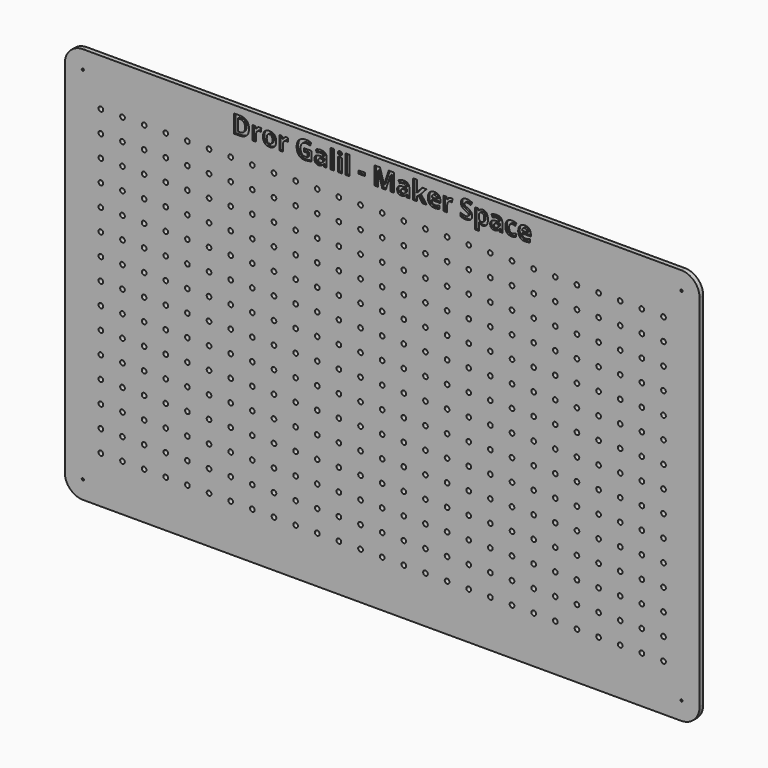
from build123d import *

# Parameters (mm, degrees)
F0_W         = 880
F0_H         = 550
F0_R         = 3.25
F1_DEPTH     = 6.35
F2_R         = 1.5
F3_DEPTH     = 25
F4_R         = 25.4
F5_TEXT_SIZE = 34.7222222222
F6_DEPTH     = 2.54


# Not quite as in the source:
# - Text() gives the source's letters only with a copy of the font that has no kerning and outlines rounded to 1/6400 em; it was checked with that copy


with BuildPart() as f1:
    # F0 (on Front) → F1 (new body)
    with BuildSketch(Plane.XZ):
        Rectangle(F0_W, F0_H)
        with Locations((-390, -210)):
            Circle(F0_R, mode=Mode.SUBTRACT)
        with Locations((-360, -210)):
            Circle(F0_R, mode=Mode.SUBTRACT)
        with Locations((-330, -210)):
            Circle(F0_R, mode=Mode.SUBTRACT)
        with Locations((-300, -210)):
            Circle(F0_R, mode=Mode.SUBTRACT)
        with Locations((-270, -210)):
            Circle(F0_R, mode=Mode.SUBTRACT)
        with Locations((-240, -210)):
            Circle(F0_R, mode=Mode.SUBTRACT)
        with Locations((-390, -180)):
            Circle(F0_R, mode=Mode.SUBTRACT)
        with Locations((-360, -180)):
            Circle(F0_R, mode=Mode.SUBTRACT)
        with Locations((-390, -150)):
            Circle(F0_R, mode=Mode.SUBTRACT)
        with Locations((-360, -150)):
            Circle(F0_R, mode=Mode.SUBTRACT)
        with Locations((-330, -180)):
            Circle(F0_R, mode=Mode.SUBTRACT)
        with Locations((-300, -180)):
            Circle(F0_R, mode=Mode.SUBTRACT)
        with Locations((-270, -180)):
            Circle(F0_R, mode=Mode.SUBTRACT)
        with Locations((-240, -180)):
            Circle(F0_R, mode=Mode.SUBTRACT)
        with Locations((-330, -150)):
            Circle(F0_R, mode=Mode.SUBTRACT)
        with Locations((-300, -150)):
            Circle(F0_R, mode=Mode.SUBTRACT)
        with Locations((-270, -150)):
            Circle(F0_R, mode=Mode.SUBTRACT)
        with Locations((-240, -150)):
            Circle(F0_R, mode=Mode.SUBTRACT)
        with Locations((-210, -210)):
            Circle(F0_R, mode=Mode.SUBTRACT)
        with Locations((-180, -210)):
            Circle(F0_R, mode=Mode.SUBTRACT)
        with Locations((-150, -210)):
            Circle(F0_R, mode=Mode.SUBTRACT)
        with Locations((-120, -210)):
            Circle(F0_R, mode=Mode.SUBTRACT)
        with Locations((-90, -210)):
            Circle(F0_R, mode=Mode.SUBTRACT)
        with Locations((-60, -210)):
            Circle(F0_R, mode=Mode.SUBTRACT)
        with Locations((-30, -210)):
            Circle(F0_R, mode=Mode.SUBTRACT)
        with Locations((-210, -180)):
            Circle(F0_R, mode=Mode.SUBTRACT)
        with Locations((-180, -180)):
            Circle(F0_R, mode=Mode.SUBTRACT)
        with Locations((-150, -180)):
            Circle(F0_R, mode=Mode.SUBTRACT)
        with Locations((-120, -180)):
            Circle(F0_R, mode=Mode.SUBTRACT)
        with Locations((-210, -150)):
            Circle(F0_R, mode=Mode.SUBTRACT)
        with Locations((-180, -150)):
            Circle(F0_R, mode=Mode.SUBTRACT)
        with Locations((-150, -150)):
            Circle(F0_R, mode=Mode.SUBTRACT)
        with Locations((-120, -150)):
            Circle(F0_R, mode=Mode.SUBTRACT)
        with Locations((-90, -180)):
            Circle(F0_R, mode=Mode.SUBTRACT)
        with Locations((-60, -180)):
            Circle(F0_R, mode=Mode.SUBTRACT)
        with Locations((-30, -180)):
            Circle(F0_R, mode=Mode.SUBTRACT)
        with Locations((-90, -150)):
            Circle(F0_R, mode=Mode.SUBTRACT)
        with Locations((-60, -150)):
            Circle(F0_R, mode=Mode.SUBTRACT)
        with Locations((-30, -150)):
            Circle(F0_R, mode=Mode.SUBTRACT)
        with Locations((-390, -120)):
            Circle(F0_R, mode=Mode.SUBTRACT)
        with Locations((-360, -120)):
            Circle(F0_R, mode=Mode.SUBTRACT)
        with Locations((-390, -90)):
            Circle(F0_R, mode=Mode.SUBTRACT)
        with Locations((-360, -90)):
            Circle(F0_R, mode=Mode.SUBTRACT)
        with Locations((-330, -120)):
            Circle(F0_R, mode=Mode.SUBTRACT)
        with Locations((-300, -120)):
            Circle(F0_R, mode=Mode.SUBTRACT)
        with Locations((-270, -120)):
            Circle(F0_R, mode=Mode.SUBTRACT)
        with Locations((-240, -120)):
            Circle(F0_R, mode=Mode.SUBTRACT)
        with Locations((-330, -90)):
            Circle(F0_R, mode=Mode.SUBTRACT)
        with Locations((-300, -90)):
            Circle(F0_R, mode=Mode.SUBTRACT)
        with Locations((-270, -90)):
            Circle(F0_R, mode=Mode.SUBTRACT)
        with Locations((-240, -90)):
            Circle(F0_R, mode=Mode.SUBTRACT)
        with Locations((-390, -60)):
            Circle(F0_R, mode=Mode.SUBTRACT)
        with Locations((-360, -60)):
            Circle(F0_R, mode=Mode.SUBTRACT)
        with Locations((-390, -30)):
            Circle(F0_R, mode=Mode.SUBTRACT)
        with Locations((-360, -30)):
            Circle(F0_R, mode=Mode.SUBTRACT)
        with Locations((-330, -60)):
            Circle(F0_R, mode=Mode.SUBTRACT)
        with Locations((-300, -60)):
            Circle(F0_R, mode=Mode.SUBTRACT)
        with Locations((-270, -60)):
            Circle(F0_R, mode=Mode.SUBTRACT)
        with Locations((-240, -60)):
            Circle(F0_R, mode=Mode.SUBTRACT)
        with Locations((-330, -30)):
            Circle(F0_R, mode=Mode.SUBTRACT)
        with Locations((-300, -30)):
            Circle(F0_R, mode=Mode.SUBTRACT)
        with Locations((-270, -30)):
            Circle(F0_R, mode=Mode.SUBTRACT)
        with Locations((-240, -30)):
            Circle(F0_R, mode=Mode.SUBTRACT)
        with Locations((-210, -120)):
            Circle(F0_R, mode=Mode.SUBTRACT)
        with Locations((-180, -120)):
            Circle(F0_R, mode=Mode.SUBTRACT)
        with Locations((-150, -120)):
            Circle(F0_R, mode=Mode.SUBTRACT)
        with Locations((-120, -120)):
            Circle(F0_R, mode=Mode.SUBTRACT)
        with Locations((-210, -90)):
            Circle(F0_R, mode=Mode.SUBTRACT)
        with Locations((-180, -90)):
            Circle(F0_R, mode=Mode.SUBTRACT)
        with Locations((-150, -90)):
            Circle(F0_R, mode=Mode.SUBTRACT)
        with Locations((-120, -90)):
            Circle(F0_R, mode=Mode.SUBTRACT)
        with Locations((-90, -120)):
            Circle(F0_R, mode=Mode.SUBTRACT)
        with Locations((-60, -120)):
            Circle(F0_R, mode=Mode.SUBTRACT)
        with Locations((-30, -120)):
            Circle(F0_R, mode=Mode.SUBTRACT)
        with Locations((-90, -90)):
            Circle(F0_R, mode=Mode.SUBTRACT)
        with Locations((-60, -90)):
            Circle(F0_R, mode=Mode.SUBTRACT)
        with Locations((-30, -90)):
            Circle(F0_R, mode=Mode.SUBTRACT)
        with Locations((-210, -60)):
            Circle(F0_R, mode=Mode.SUBTRACT)
        with Locations((-180, -60)):
            Circle(F0_R, mode=Mode.SUBTRACT)
        with Locations((-150, -60)):
            Circle(F0_R, mode=Mode.SUBTRACT)
        with Locations((-120, -60)):
            Circle(F0_R, mode=Mode.SUBTRACT)
        with Locations((-210, -30)):
            Circle(F0_R, mode=Mode.SUBTRACT)
        with Locations((-180, -30)):
            Circle(F0_R, mode=Mode.SUBTRACT)
        with Locations((-150, -30)):
            Circle(F0_R, mode=Mode.SUBTRACT)
        with Locations((-120, -30)):
            Circle(F0_R, mode=Mode.SUBTRACT)
        with Locations((-90, -60)):
            Circle(F0_R, mode=Mode.SUBTRACT)
        with Locations((-60, -60)):
            Circle(F0_R, mode=Mode.SUBTRACT)
        with Locations((-30, -60)):
            Circle(F0_R, mode=Mode.SUBTRACT)
        with Locations((-90, -30)):
            Circle(F0_R, mode=Mode.SUBTRACT)
        with Locations((-60, -30)):
            Circle(F0_R, mode=Mode.SUBTRACT)
        with Locations((-30, -30)):
            Circle(F0_R, mode=Mode.SUBTRACT)
        with Locations((0, -210)):
            Circle(F0_R, mode=Mode.SUBTRACT)
        with Locations((30, -210)):
            Circle(F0_R, mode=Mode.SUBTRACT)
        with Locations((60, -210)):
            Circle(F0_R, mode=Mode.SUBTRACT)
        with Locations((90, -210)):
            Circle(F0_R, mode=Mode.SUBTRACT)
        with Locations((120, -210)):
            Circle(F0_R, mode=Mode.SUBTRACT)
        with Locations((150, -210)):
            Circle(F0_R, mode=Mode.SUBTRACT)
        with Locations((180, -210)):
            Circle(F0_R, mode=Mode.SUBTRACT)
        with Locations((210, -210)):
            Circle(F0_R, mode=Mode.SUBTRACT)
        with Locations((0, -180)):
            Circle(F0_R, mode=Mode.SUBTRACT)
        with Locations((30, -180)):
            Circle(F0_R, mode=Mode.SUBTRACT)
        with Locations((60, -180)):
            Circle(F0_R, mode=Mode.SUBTRACT)
        with Locations((90, -180)):
            Circle(F0_R, mode=Mode.SUBTRACT)
        with Locations((0, -150)):
            Circle(F0_R, mode=Mode.SUBTRACT)
        with Locations((30, -150)):
            Circle(F0_R, mode=Mode.SUBTRACT)
        with Locations((60, -150)):
            Circle(F0_R, mode=Mode.SUBTRACT)
        with Locations((90, -150)):
            Circle(F0_R, mode=Mode.SUBTRACT)
        with Locations((120, -180)):
            Circle(F0_R, mode=Mode.SUBTRACT)
        with Locations((150, -180)):
            Circle(F0_R, mode=Mode.SUBTRACT)
        with Locations((180, -180)):
            Circle(F0_R, mode=Mode.SUBTRACT)
        with Locations((210, -180)):
            Circle(F0_R, mode=Mode.SUBTRACT)
        with Locations((120, -150)):
            Circle(F0_R, mode=Mode.SUBTRACT)
        with Locations((150, -150)):
            Circle(F0_R, mode=Mode.SUBTRACT)
        with Locations((180, -150)):
            Circle(F0_R, mode=Mode.SUBTRACT)
        with Locations((210, -150)):
            Circle(F0_R, mode=Mode.SUBTRACT)
        with Locations((240, -210)):
            Circle(F0_R, mode=Mode.SUBTRACT)
        with Locations((270, -210)):
            Circle(F0_R, mode=Mode.SUBTRACT)
        with Locations((300, -210)):
            Circle(F0_R, mode=Mode.SUBTRACT)
        with Locations((330, -210)):
            Circle(F0_R, mode=Mode.SUBTRACT)
        with Locations((360, -210)):
            Circle(F0_R, mode=Mode.SUBTRACT)
        with Locations((390, -210)):
            Circle(F0_R, mode=Mode.SUBTRACT)
        with Locations((240, -180)):
            Circle(F0_R, mode=Mode.SUBTRACT)
        with Locations((270, -180)):
            Circle(F0_R, mode=Mode.SUBTRACT)
        with Locations((300, -180)):
            Circle(F0_R, mode=Mode.SUBTRACT)
        with Locations((240, -150)):
            Circle(F0_R, mode=Mode.SUBTRACT)
        with Locations((270, -150)):
            Circle(F0_R, mode=Mode.SUBTRACT)
        with Locations((300, -150)):
            Circle(F0_R, mode=Mode.SUBTRACT)
        with Locations((330, -180)):
            Circle(F0_R, mode=Mode.SUBTRACT)
        with Locations((360, -180)):
            Circle(F0_R, mode=Mode.SUBTRACT)
        with Locations((390, -180)):
            Circle(F0_R, mode=Mode.SUBTRACT)
        with Locations((330, -150)):
            Circle(F0_R, mode=Mode.SUBTRACT)
        with Locations((360, -150)):
            Circle(F0_R, mode=Mode.SUBTRACT)
        with Locations((390, -150)):
            Circle(F0_R, mode=Mode.SUBTRACT)
        with Locations((0, -120)):
            Circle(F0_R, mode=Mode.SUBTRACT)
        with Locations((30, -120)):
            Circle(F0_R, mode=Mode.SUBTRACT)
        with Locations((60, -120)):
            Circle(F0_R, mode=Mode.SUBTRACT)
        with Locations((90, -120)):
            Circle(F0_R, mode=Mode.SUBTRACT)
        with Locations((0, -90)):
            Circle(F0_R, mode=Mode.SUBTRACT)
        with Locations((30, -90)):
            Circle(F0_R, mode=Mode.SUBTRACT)
        with Locations((60, -90)):
            Circle(F0_R, mode=Mode.SUBTRACT)
        with Locations((90, -90)):
            Circle(F0_R, mode=Mode.SUBTRACT)
        with Locations((120, -120)):
            Circle(F0_R, mode=Mode.SUBTRACT)
        with Locations((150, -120)):
            Circle(F0_R, mode=Mode.SUBTRACT)
        with Locations((180, -120)):
            Circle(F0_R, mode=Mode.SUBTRACT)
        with Locations((210, -120)):
            Circle(F0_R, mode=Mode.SUBTRACT)
        with Locations((120, -90)):
            Circle(F0_R, mode=Mode.SUBTRACT)
        with Locations((150, -90)):
            Circle(F0_R, mode=Mode.SUBTRACT)
        with Locations((180, -90)):
            Circle(F0_R, mode=Mode.SUBTRACT)
        with Locations((210, -90)):
            Circle(F0_R, mode=Mode.SUBTRACT)
        with Locations((0, -60)):
            Circle(F0_R, mode=Mode.SUBTRACT)
        with Locations((30, -60)):
            Circle(F0_R, mode=Mode.SUBTRACT)
        with Locations((60, -60)):
            Circle(F0_R, mode=Mode.SUBTRACT)
        with Locations((90, -60)):
            Circle(F0_R, mode=Mode.SUBTRACT)
        with Locations((0, -30)):
            Circle(F0_R, mode=Mode.SUBTRACT)
        with Locations((30, -30)):
            Circle(F0_R, mode=Mode.SUBTRACT)
        with Locations((60, -30)):
            Circle(F0_R, mode=Mode.SUBTRACT)
        with Locations((90, -30)):
            Circle(F0_R, mode=Mode.SUBTRACT)
        with Locations((120, -60)):
            Circle(F0_R, mode=Mode.SUBTRACT)
        with Locations((150, -60)):
            Circle(F0_R, mode=Mode.SUBTRACT)
        with Locations((180, -60)):
            Circle(F0_R, mode=Mode.SUBTRACT)
        with Locations((210, -60)):
            Circle(F0_R, mode=Mode.SUBTRACT)
        with Locations((120, -30)):
            Circle(F0_R, mode=Mode.SUBTRACT)
        with Locations((150, -30)):
            Circle(F0_R, mode=Mode.SUBTRACT)
        with Locations((180, -30)):
            Circle(F0_R, mode=Mode.SUBTRACT)
        with Locations((210, -30)):
            Circle(F0_R, mode=Mode.SUBTRACT)
        with Locations((240, -120)):
            Circle(F0_R, mode=Mode.SUBTRACT)
        with Locations((270, -120)):
            Circle(F0_R, mode=Mode.SUBTRACT)
        with Locations((300, -120)):
            Circle(F0_R, mode=Mode.SUBTRACT)
        with Locations((240, -90)):
            Circle(F0_R, mode=Mode.SUBTRACT)
        with Locations((270, -90)):
            Circle(F0_R, mode=Mode.SUBTRACT)
        with Locations((300, -90)):
            Circle(F0_R, mode=Mode.SUBTRACT)
        with Locations((330, -120)):
            Circle(F0_R, mode=Mode.SUBTRACT)
        with Locations((360, -120)):
            Circle(F0_R, mode=Mode.SUBTRACT)
        with Locations((390, -120)):
            Circle(F0_R, mode=Mode.SUBTRACT)
        with Locations((330, -90)):
            Circle(F0_R, mode=Mode.SUBTRACT)
        with Locations((360, -90)):
            Circle(F0_R, mode=Mode.SUBTRACT)
        with Locations((390, -90)):
            Circle(F0_R, mode=Mode.SUBTRACT)
        with Locations((240, -60)):
            Circle(F0_R, mode=Mode.SUBTRACT)
        with Locations((270, -60)):
            Circle(F0_R, mode=Mode.SUBTRACT)
        with Locations((300, -60)):
            Circle(F0_R, mode=Mode.SUBTRACT)
        with Locations((240, -30)):
            Circle(F0_R, mode=Mode.SUBTRACT)
        with Locations((270, -30)):
            Circle(F0_R, mode=Mode.SUBTRACT)
        with Locations((300, -30)):
            Circle(F0_R, mode=Mode.SUBTRACT)
        with Locations((330, -60)):
            Circle(F0_R, mode=Mode.SUBTRACT)
        with Locations((360, -60)):
            Circle(F0_R, mode=Mode.SUBTRACT)
        with Locations((390, -60)):
            Circle(F0_R, mode=Mode.SUBTRACT)
        with Locations((330, -30)):
            Circle(F0_R, mode=Mode.SUBTRACT)
        with Locations((360, -30)):
            Circle(F0_R, mode=Mode.SUBTRACT)
        with Locations((390, -30)):
            Circle(F0_R, mode=Mode.SUBTRACT)
        with Locations((-390, 0)):
            Circle(F0_R, mode=Mode.SUBTRACT)
        with Locations((-390, 30)):
            Circle(F0_R, mode=Mode.SUBTRACT)
        with Locations((-360, 0)):
            Circle(F0_R, mode=Mode.SUBTRACT)
        with Locations((-360, 30)):
            Circle(F0_R, mode=Mode.SUBTRACT)
        with Locations((-390, 60)):
            Circle(F0_R, mode=Mode.SUBTRACT)
        with Locations((-360, 60)):
            Circle(F0_R, mode=Mode.SUBTRACT)
        with Locations((-330, 0)):
            Circle(F0_R, mode=Mode.SUBTRACT)
        with Locations((-300, 0)):
            Circle(F0_R, mode=Mode.SUBTRACT)
        with Locations((-330, 30)):
            Circle(F0_R, mode=Mode.SUBTRACT)
        with Locations((-300, 30)):
            Circle(F0_R, mode=Mode.SUBTRACT)
        with Locations((-270, 0)):
            Circle(F0_R, mode=Mode.SUBTRACT)
        with Locations((-240, 0)):
            Circle(F0_R, mode=Mode.SUBTRACT)
        with Locations((-270, 30)):
            Circle(F0_R, mode=Mode.SUBTRACT)
        with Locations((-240, 30)):
            Circle(F0_R, mode=Mode.SUBTRACT)
        with Locations((-330, 60)):
            Circle(F0_R, mode=Mode.SUBTRACT)
        with Locations((-300, 60)):
            Circle(F0_R, mode=Mode.SUBTRACT)
        with Locations((-270, 60)):
            Circle(F0_R, mode=Mode.SUBTRACT)
        with Locations((-240, 60)):
            Circle(F0_R, mode=Mode.SUBTRACT)
        with Locations((-390, 90)):
            Circle(F0_R, mode=Mode.SUBTRACT)
        with Locations((-360, 90)):
            Circle(F0_R, mode=Mode.SUBTRACT)
        with Locations((-390, 120)):
            Circle(F0_R, mode=Mode.SUBTRACT)
        with Locations((-360, 120)):
            Circle(F0_R, mode=Mode.SUBTRACT)
        with Locations((-330, 90)):
            Circle(F0_R, mode=Mode.SUBTRACT)
        with Locations((-300, 90)):
            Circle(F0_R, mode=Mode.SUBTRACT)
        with Locations((-270, 90)):
            Circle(F0_R, mode=Mode.SUBTRACT)
        with Locations((-240, 90)):
            Circle(F0_R, mode=Mode.SUBTRACT)
        with Locations((-330, 120)):
            Circle(F0_R, mode=Mode.SUBTRACT)
        with Locations((-300, 120)):
            Circle(F0_R, mode=Mode.SUBTRACT)
        with Locations((-270, 120)):
            Circle(F0_R, mode=Mode.SUBTRACT)
        with Locations((-240, 120)):
            Circle(F0_R, mode=Mode.SUBTRACT)
        with Locations((-210, 0)):
            Circle(F0_R, mode=Mode.SUBTRACT)
        with Locations((-180, 0)):
            Circle(F0_R, mode=Mode.SUBTRACT)
        with Locations((-210, 30)):
            Circle(F0_R, mode=Mode.SUBTRACT)
        with Locations((-180, 30)):
            Circle(F0_R, mode=Mode.SUBTRACT)
        with Locations((-150, 0)):
            Circle(F0_R, mode=Mode.SUBTRACT)
        with Locations((-120, 0)):
            Circle(F0_R, mode=Mode.SUBTRACT)
        with Locations((-150, 30)):
            Circle(F0_R, mode=Mode.SUBTRACT)
        with Locations((-120, 30)):
            Circle(F0_R, mode=Mode.SUBTRACT)
        with Locations((-210, 60)):
            Circle(F0_R, mode=Mode.SUBTRACT)
        with Locations((-180, 60)):
            Circle(F0_R, mode=Mode.SUBTRACT)
        with Locations((-150, 60)):
            Circle(F0_R, mode=Mode.SUBTRACT)
        with Locations((-120, 60)):
            Circle(F0_R, mode=Mode.SUBTRACT)
        with Locations((-90, 0)):
            Circle(F0_R, mode=Mode.SUBTRACT)
        with Locations((-60, 0)):
            Circle(F0_R, mode=Mode.SUBTRACT)
        with Locations((-90, 30)):
            Circle(F0_R, mode=Mode.SUBTRACT)
        with Locations((-60, 30)):
            Circle(F0_R, mode=Mode.SUBTRACT)
        with Locations((-30, 0)):
            Circle(F0_R, mode=Mode.SUBTRACT)
        with Locations((-30, 30)):
            Circle(F0_R, mode=Mode.SUBTRACT)
        with Locations((-90, 60)):
            Circle(F0_R, mode=Mode.SUBTRACT)
        with Locations((-60, 60)):
            Circle(F0_R, mode=Mode.SUBTRACT)
        with Locations((-30, 60)):
            Circle(F0_R, mode=Mode.SUBTRACT)
        with Locations((-210, 90)):
            Circle(F0_R, mode=Mode.SUBTRACT)
        with Locations((-180, 90)):
            Circle(F0_R, mode=Mode.SUBTRACT)
        with Locations((-150, 90)):
            Circle(F0_R, mode=Mode.SUBTRACT)
        with Locations((-120, 90)):
            Circle(F0_R, mode=Mode.SUBTRACT)
        with Locations((-210, 120)):
            Circle(F0_R, mode=Mode.SUBTRACT)
        with Locations((-180, 120)):
            Circle(F0_R, mode=Mode.SUBTRACT)
        with Locations((-150, 120)):
            Circle(F0_R, mode=Mode.SUBTRACT)
        with Locations((-120, 120)):
            Circle(F0_R, mode=Mode.SUBTRACT)
        with Locations((-90, 90)):
            Circle(F0_R, mode=Mode.SUBTRACT)
        with Locations((-60, 90)):
            Circle(F0_R, mode=Mode.SUBTRACT)
        with Locations((-30, 90)):
            Circle(F0_R, mode=Mode.SUBTRACT)
        with Locations((-90, 120)):
            Circle(F0_R, mode=Mode.SUBTRACT)
        with Locations((-60, 120)):
            Circle(F0_R, mode=Mode.SUBTRACT)
        with Locations((-30, 120)):
            Circle(F0_R, mode=Mode.SUBTRACT)
        with Locations((-390, 150)):
            Circle(F0_R, mode=Mode.SUBTRACT)
        with Locations((-360, 150)):
            Circle(F0_R, mode=Mode.SUBTRACT)
        with Locations((-390, 180)):
            Circle(F0_R, mode=Mode.SUBTRACT)
        with Locations((-360, 180)):
            Circle(F0_R, mode=Mode.SUBTRACT)
        with Locations((-330, 150)):
            Circle(F0_R, mode=Mode.SUBTRACT)
        with Locations((-300, 150)):
            Circle(F0_R, mode=Mode.SUBTRACT)
        with Locations((-270, 150)):
            Circle(F0_R, mode=Mode.SUBTRACT)
        with Locations((-240, 150)):
            Circle(F0_R, mode=Mode.SUBTRACT)
        with Locations((-330, 180)):
            Circle(F0_R, mode=Mode.SUBTRACT)
        with Locations((-300, 180)):
            Circle(F0_R, mode=Mode.SUBTRACT)
        with Locations((-270, 180)):
            Circle(F0_R, mode=Mode.SUBTRACT)
        with Locations((-240, 180)):
            Circle(F0_R, mode=Mode.SUBTRACT)
        with Locations((-390, 210)):
            Circle(F0_R, mode=Mode.SUBTRACT)
        with Locations((-360, 210)):
            Circle(F0_R, mode=Mode.SUBTRACT)
        with Locations((-330, 210)):
            Circle(F0_R, mode=Mode.SUBTRACT)
        with Locations((-300, 210)):
            Circle(F0_R, mode=Mode.SUBTRACT)
        with Locations((-270, 210)):
            Circle(F0_R, mode=Mode.SUBTRACT)
        with Locations((-240, 210)):
            Circle(F0_R, mode=Mode.SUBTRACT)
        with Locations((-210, 150)):
            Circle(F0_R, mode=Mode.SUBTRACT)
        with Locations((-180, 150)):
            Circle(F0_R, mode=Mode.SUBTRACT)
        with Locations((-150, 150)):
            Circle(F0_R, mode=Mode.SUBTRACT)
        with Locations((-120, 150)):
            Circle(F0_R, mode=Mode.SUBTRACT)
        with Locations((-210, 180)):
            Circle(F0_R, mode=Mode.SUBTRACT)
        with Locations((-180, 180)):
            Circle(F0_R, mode=Mode.SUBTRACT)
        with Locations((-150, 180)):
            Circle(F0_R, mode=Mode.SUBTRACT)
        with Locations((-120, 180)):
            Circle(F0_R, mode=Mode.SUBTRACT)
        with Locations((-90, 150)):
            Circle(F0_R, mode=Mode.SUBTRACT)
        with Locations((-60, 150)):
            Circle(F0_R, mode=Mode.SUBTRACT)
        with Locations((-30, 150)):
            Circle(F0_R, mode=Mode.SUBTRACT)
        with Locations((-90, 180)):
            Circle(F0_R, mode=Mode.SUBTRACT)
        with Locations((-60, 180)):
            Circle(F0_R, mode=Mode.SUBTRACT)
        with Locations((-30, 180)):
            Circle(F0_R, mode=Mode.SUBTRACT)
        with Locations((-210, 210)):
            Circle(F0_R, mode=Mode.SUBTRACT)
        with Locations((-180, 210)):
            Circle(F0_R, mode=Mode.SUBTRACT)
        with Locations((-150, 210)):
            Circle(F0_R, mode=Mode.SUBTRACT)
        with Locations((-120, 210)):
            Circle(F0_R, mode=Mode.SUBTRACT)
        with Locations((-90, 210)):
            Circle(F0_R, mode=Mode.SUBTRACT)
        with Locations((-60, 210)):
            Circle(F0_R, mode=Mode.SUBTRACT)
        with Locations((-30, 210)):
            Circle(F0_R, mode=Mode.SUBTRACT)
        Circle(F0_R, mode=Mode.SUBTRACT)
        with Locations((30, 0)):
            Circle(F0_R, mode=Mode.SUBTRACT)
        with Locations((0, 30)):
            Circle(F0_R, mode=Mode.SUBTRACT)
        with Locations((30, 30)):
            Circle(F0_R, mode=Mode.SUBTRACT)
        with Locations((60, 0)):
            Circle(F0_R, mode=Mode.SUBTRACT)
        with Locations((90, 0)):
            Circle(F0_R, mode=Mode.SUBTRACT)
        with Locations((60, 30)):
            Circle(F0_R, mode=Mode.SUBTRACT)
        with Locations((90, 30)):
            Circle(F0_R, mode=Mode.SUBTRACT)
        with Locations((0, 60)):
            Circle(F0_R, mode=Mode.SUBTRACT)
        with Locations((30, 60)):
            Circle(F0_R, mode=Mode.SUBTRACT)
        with Locations((60, 60)):
            Circle(F0_R, mode=Mode.SUBTRACT)
        with Locations((90, 60)):
            Circle(F0_R, mode=Mode.SUBTRACT)
        with Locations((120, 0)):
            Circle(F0_R, mode=Mode.SUBTRACT)
        with Locations((150, 0)):
            Circle(F0_R, mode=Mode.SUBTRACT)
        with Locations((120, 30)):
            Circle(F0_R, mode=Mode.SUBTRACT)
        with Locations((150, 30)):
            Circle(F0_R, mode=Mode.SUBTRACT)
        with Locations((180, 0)):
            Circle(F0_R, mode=Mode.SUBTRACT)
        with Locations((210, 0)):
            Circle(F0_R, mode=Mode.SUBTRACT)
        with Locations((180, 30)):
            Circle(F0_R, mode=Mode.SUBTRACT)
        with Locations((210, 30)):
            Circle(F0_R, mode=Mode.SUBTRACT)
        with Locations((120, 60)):
            Circle(F0_R, mode=Mode.SUBTRACT)
        with Locations((150, 60)):
            Circle(F0_R, mode=Mode.SUBTRACT)
        with Locations((180, 60)):
            Circle(F0_R, mode=Mode.SUBTRACT)
        with Locations((210, 60)):
            Circle(F0_R, mode=Mode.SUBTRACT)
        with Locations((0, 90)):
            Circle(F0_R, mode=Mode.SUBTRACT)
        with Locations((30, 90)):
            Circle(F0_R, mode=Mode.SUBTRACT)
        with Locations((60, 90)):
            Circle(F0_R, mode=Mode.SUBTRACT)
        with Locations((90, 90)):
            Circle(F0_R, mode=Mode.SUBTRACT)
        with Locations((0, 120)):
            Circle(F0_R, mode=Mode.SUBTRACT)
        with Locations((30, 120)):
            Circle(F0_R, mode=Mode.SUBTRACT)
        with Locations((60, 120)):
            Circle(F0_R, mode=Mode.SUBTRACT)
        with Locations((90, 120)):
            Circle(F0_R, mode=Mode.SUBTRACT)
        with Locations((120, 90)):
            Circle(F0_R, mode=Mode.SUBTRACT)
        with Locations((150, 90)):
            Circle(F0_R, mode=Mode.SUBTRACT)
        with Locations((180, 90)):
            Circle(F0_R, mode=Mode.SUBTRACT)
        with Locations((210, 90)):
            Circle(F0_R, mode=Mode.SUBTRACT)
        with Locations((120, 120)):
            Circle(F0_R, mode=Mode.SUBTRACT)
        with Locations((150, 120)):
            Circle(F0_R, mode=Mode.SUBTRACT)
        with Locations((180, 120)):
            Circle(F0_R, mode=Mode.SUBTRACT)
        with Locations((210, 120)):
            Circle(F0_R, mode=Mode.SUBTRACT)
        with Locations((240, 0)):
            Circle(F0_R, mode=Mode.SUBTRACT)
        with Locations((270, 0)):
            Circle(F0_R, mode=Mode.SUBTRACT)
        with Locations((240, 30)):
            Circle(F0_R, mode=Mode.SUBTRACT)
        with Locations((270, 30)):
            Circle(F0_R, mode=Mode.SUBTRACT)
        with Locations((300, 0)):
            Circle(F0_R, mode=Mode.SUBTRACT)
        with Locations((300, 30)):
            Circle(F0_R, mode=Mode.SUBTRACT)
        with Locations((240, 60)):
            Circle(F0_R, mode=Mode.SUBTRACT)
        with Locations((270, 60)):
            Circle(F0_R, mode=Mode.SUBTRACT)
        with Locations((300, 60)):
            Circle(F0_R, mode=Mode.SUBTRACT)
        with Locations((330, 0)):
            Circle(F0_R, mode=Mode.SUBTRACT)
        with Locations((360, 0)):
            Circle(F0_R, mode=Mode.SUBTRACT)
        with Locations((330, 30)):
            Circle(F0_R, mode=Mode.SUBTRACT)
        with Locations((360, 30)):
            Circle(F0_R, mode=Mode.SUBTRACT)
        with Locations((390, 0)):
            Circle(F0_R, mode=Mode.SUBTRACT)
        with Locations((390, 30)):
            Circle(F0_R, mode=Mode.SUBTRACT)
        with Locations((330, 60)):
            Circle(F0_R, mode=Mode.SUBTRACT)
        with Locations((360, 60)):
            Circle(F0_R, mode=Mode.SUBTRACT)
        with Locations((390, 60)):
            Circle(F0_R, mode=Mode.SUBTRACT)
        with Locations((240, 90)):
            Circle(F0_R, mode=Mode.SUBTRACT)
        with Locations((270, 90)):
            Circle(F0_R, mode=Mode.SUBTRACT)
        with Locations((300, 90)):
            Circle(F0_R, mode=Mode.SUBTRACT)
        with Locations((240, 120)):
            Circle(F0_R, mode=Mode.SUBTRACT)
        with Locations((270, 120)):
            Circle(F0_R, mode=Mode.SUBTRACT)
        with Locations((300, 120)):
            Circle(F0_R, mode=Mode.SUBTRACT)
        with Locations((330, 90)):
            Circle(F0_R, mode=Mode.SUBTRACT)
        with Locations((360, 90)):
            Circle(F0_R, mode=Mode.SUBTRACT)
        with Locations((390, 90)):
            Circle(F0_R, mode=Mode.SUBTRACT)
        with Locations((330, 120)):
            Circle(F0_R, mode=Mode.SUBTRACT)
        with Locations((360, 120)):
            Circle(F0_R, mode=Mode.SUBTRACT)
        with Locations((390, 120)):
            Circle(F0_R, mode=Mode.SUBTRACT)
        with Locations((0, 150)):
            Circle(F0_R, mode=Mode.SUBTRACT)
        with Locations((30, 150)):
            Circle(F0_R, mode=Mode.SUBTRACT)
        with Locations((60, 150)):
            Circle(F0_R, mode=Mode.SUBTRACT)
        with Locations((90, 150)):
            Circle(F0_R, mode=Mode.SUBTRACT)
        with Locations((0, 180)):
            Circle(F0_R, mode=Mode.SUBTRACT)
        with Locations((30, 180)):
            Circle(F0_R, mode=Mode.SUBTRACT)
        with Locations((60, 180)):
            Circle(F0_R, mode=Mode.SUBTRACT)
        with Locations((90, 180)):
            Circle(F0_R, mode=Mode.SUBTRACT)
        with Locations((120, 150)):
            Circle(F0_R, mode=Mode.SUBTRACT)
        with Locations((150, 150)):
            Circle(F0_R, mode=Mode.SUBTRACT)
        with Locations((180, 150)):
            Circle(F0_R, mode=Mode.SUBTRACT)
        with Locations((210, 150)):
            Circle(F0_R, mode=Mode.SUBTRACT)
        with Locations((120, 180)):
            Circle(F0_R, mode=Mode.SUBTRACT)
        with Locations((150, 180)):
            Circle(F0_R, mode=Mode.SUBTRACT)
        with Locations((180, 180)):
            Circle(F0_R, mode=Mode.SUBTRACT)
        with Locations((210, 180)):
            Circle(F0_R, mode=Mode.SUBTRACT)
        with Locations((0, 210)):
            Circle(F0_R, mode=Mode.SUBTRACT)
        with Locations((30, 210)):
            Circle(F0_R, mode=Mode.SUBTRACT)
        with Locations((60, 210)):
            Circle(F0_R, mode=Mode.SUBTRACT)
        with Locations((90, 210)):
            Circle(F0_R, mode=Mode.SUBTRACT)
        with Locations((120, 210)):
            Circle(F0_R, mode=Mode.SUBTRACT)
        with Locations((150, 210)):
            Circle(F0_R, mode=Mode.SUBTRACT)
        with Locations((180, 210)):
            Circle(F0_R, mode=Mode.SUBTRACT)
        with Locations((210, 210)):
            Circle(F0_R, mode=Mode.SUBTRACT)
        with Locations((240, 150)):
            Circle(F0_R, mode=Mode.SUBTRACT)
        with Locations((270, 150)):
            Circle(F0_R, mode=Mode.SUBTRACT)
        with Locations((300, 150)):
            Circle(F0_R, mode=Mode.SUBTRACT)
        with Locations((240, 180)):
            Circle(F0_R, mode=Mode.SUBTRACT)
        with Locations((270, 180)):
            Circle(F0_R, mode=Mode.SUBTRACT)
        with Locations((300, 180)):
            Circle(F0_R, mode=Mode.SUBTRACT)
        with Locations((330, 150)):
            Circle(F0_R, mode=Mode.SUBTRACT)
        with Locations((360, 150)):
            Circle(F0_R, mode=Mode.SUBTRACT)
        with Locations((390, 150)):
            Circle(F0_R, mode=Mode.SUBTRACT)
        with Locations((330, 180)):
            Circle(F0_R, mode=Mode.SUBTRACT)
        with Locations((360, 180)):
            Circle(F0_R, mode=Mode.SUBTRACT)
        with Locations((390, 180)):
            Circle(F0_R, mode=Mode.SUBTRACT)
        with Locations((240, 210)):
            Circle(F0_R, mode=Mode.SUBTRACT)
        with Locations((270, 210)):
            Circle(F0_R, mode=Mode.SUBTRACT)
        with Locations((300, 210)):
            Circle(F0_R, mode=Mode.SUBTRACT)
        with Locations((330, 210)):
            Circle(F0_R, mode=Mode.SUBTRACT)
        with Locations((360, 210)):
            Circle(F0_R, mode=Mode.SUBTRACT)
        with Locations((390, 210)):
            Circle(F0_R, mode=Mode.SUBTRACT)
    extrude(amount=F1_DEPTH)

    # F2 (on face) → F3 (cut)
    with BuildSketch(Plane.XZ.offset(6.35)):
        with Locations((-415, 250)):
            Circle(F2_R)
        with Locations((415, 250)):
            Circle(F2_R)
        with Locations((415, -250)):
            Circle(F2_R)
        with Locations((-415, -250)):
            Circle(F2_R)
    extrude(amount=-F3_DEPTH, mode=Mode.SUBTRACT)

    # F4
    f4_edges = [f1.edges().sort_by_distance(p)[0] for p in [
        (-440, -3.175, 275),
        (440, -3.175, 275),
        (440, -3.175, -275),
        (-440, -3.175, -275),
    ]]
    fillet(f4_edges, radius=F4_R)

    # F5 (on face) → F6 (cut)
    with BuildSketch(Plane.XZ.offset(6.35)):
        with Locations((-208.3116319444, 240)):
            Text('Dror Galil - Maker Space', F5_TEXT_SIZE, font='Open Sans', font_style=FontStyle.BOLD, text_align=(TextAlign.LEFT, TextAlign.BOTTOM))
    extrude(amount=-F6_DEPTH, mode=Mode.SUBTRACT)


solid = f1.part
